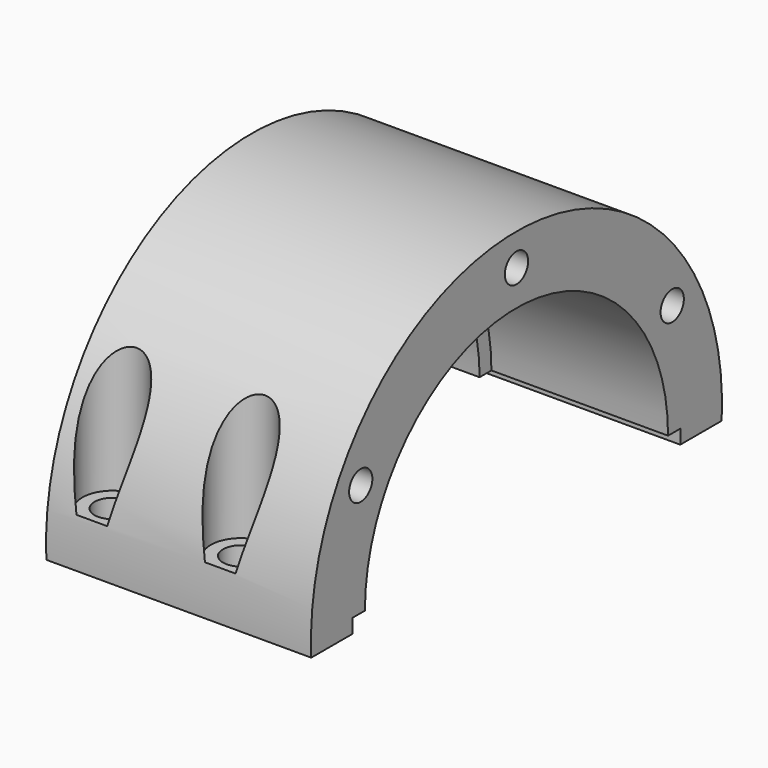
from build123d import *

# Parameters (mm, degrees)
F0_R           = 101.6
F1_DEPTH       = 104.775
F3_D           = 88.9
F3_CBORE_D     = 138.176
F3_CBORE_DEPTH = 92.075
F4_R           = 74.93
F5_DEPTH       = 69.85
F6_W           = 288.5075062513
F6_H           = 97.8503401275
F7_DEPTH       = 104.776
F8_W           = 80.9625
F8_H           = 28.0255991966
F9_DEPTH       = 104.776
F11_D          = 14.2875
F13_R          = 11.938
F14_DEPTH      = 88.1390001
F16_D          = 11.50874
F16_DEPTH      = 25.4
F16_TIP        = 3.4575743203


# Not quite as in the source:
# - a length typed as a fraction of an inch, garbled in the dataset ("3 / 203.2 mm" for 3/8 in), is restored


with BuildPart() as f1:
    # F0 (on Right) → F1 (new body)
    with BuildSketch(Plane.YZ):
        Circle(F0_R)
    extrude(amount=-F1_DEPTH)

    # F3 (through all)
    with Locations(Plane.YZ):
        with Locations((0, 0)):
            CounterBoreHole(F3_D / 2, F3_CBORE_D / 2, F3_CBORE_DEPTH)

    # F4 (on face) → F5 (cut)
    with BuildSketch(Plane.YZ):
        Circle(F4_R)
    extrude(amount=-F5_DEPTH, mode=Mode.SUBTRACT)

    # F6 (on face) → F7 (cut, through all)
    with BuildSketch(Plane.YZ):
        with Locations((9.2829242349, -54.5131700637)):
            Rectangle(F6_W, F6_H)
    extrude(amount=-F7_DEPTH, mode=Mode.SUBTRACT)

    # F8 (on face) → F9 (cut, through all)
    with BuildSketch(Plane.YZ):
        with Locations((-40.48125, -14.0127995983)):
            Rectangle(F8_W, F8_H)
        with Locations((40.48125, -14.0127995983)):
            Rectangle(F8_W, F8_H)
    extrude(amount=-F9_DEPTH, mode=Mode.SUBTRACT)

    # F11 (through all)
    with Locations(Plane(origin=(0, 0, -5.588), x_dir=(1, 0, 0), z_dir=(0, 0, -1))):
        with Locations((-36.576, 90.424), (-87.376, 90.424), (-36.576, -90.424), (-87.376, -90.424)):
            Hole(F11_D / 2)

    # F13 (on offset) → F14 (cut, through all)
    with BuildSketch(Plane(origin=(0, 0, 13.462), x_dir=(1, 0, 0), z_dir=(0, 0, -1))):
        with Locations((-87.376, 90.424)):
            Circle(F13_R)
        with Locations((-36.576, 90.424)):
            Circle(F13_R)
        with Locations((-87.376, -90.424)):
            Circle(F13_R)
        with Locations((-36.576, -90.424)):
            Circle(F13_R)
    extrude(amount=-F14_DEPTH, mode=Mode.SUBTRACT)

    # F16
    with Locations(Plane.YZ):
        with Locations((-76.9896583964, 44.45), (0, 88.9), (76.9896583964, 44.45)):
            Hole(F16_D / 2, depth=F16_DEPTH)
            with Locations((0, 0, -(F16_DEPTH + F16_TIP / 2))):  # 118° drill point
                Cone(0, F16_D / 2, F16_TIP, mode=Mode.SUBTRACT)


solid = f1.part
